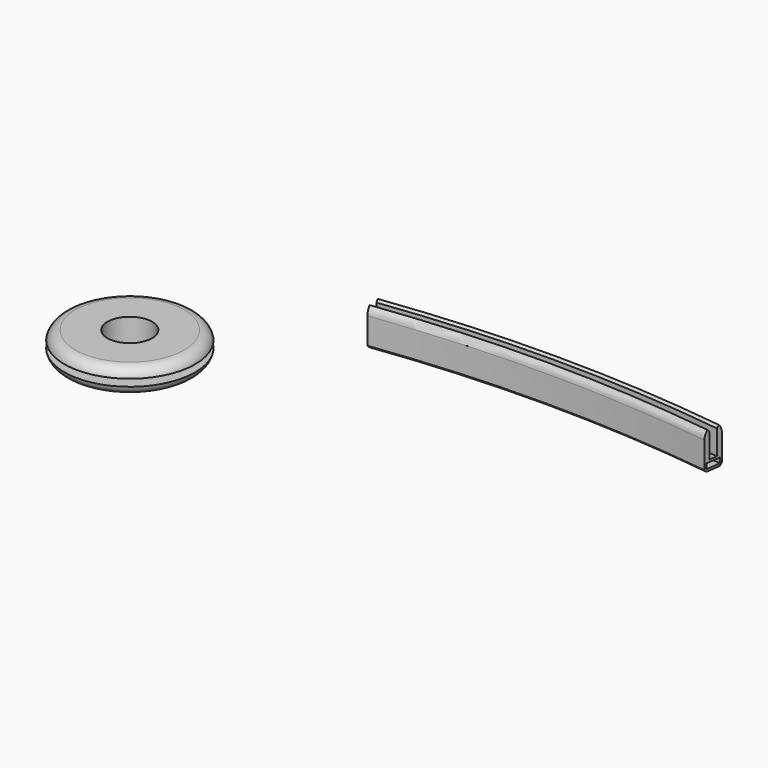
from build123d import *

# Parameters (mm, degrees)
F1_DEPTH    = 1
F4_DEPTH    = 1
F6_DEPTH    = 12
F7_SIZE     = 1
F8_T2_ANGLE = 16.6478295889
F8_T4_ANGLE = 16.6225349948
F11_SIZE    = 1
F12_R       = 22
F12_R_2     = 10
F13_DEPTH   = 3.175
F14_R       = 29.2671438264
F15_DEPTH   = 4
F17_DEPTH   = 25
F18_R       = 29.2671438264
F18_R_2     = 10
F19_DEPTH   = 4
F21_R       = 18.8886705246
F21_R_2     = 17.8886705246
F22_DEPTH   = 8


# Not quite as in the source:
# - a fillet or chamfer that OpenCascade refuses, or shapes differently, is made with other operations: its cross-section is extruded or revolved along the edge and cut away or added


with BuildPart() as f1:
    # F0 (on Top) → F1 (new body)
    with BuildSketch(Plane.XY):
        Polygon((76.2, -1.75), (76.2, 1.75), (76.2, 6.1025535688), (-76.2, 6.1025535688), (-76.2, 1.75), (-76.2, -1.75), (-76.2, -6.1025535688), (76.2, -6.1025535688), align=None)
    extrude(amount=-F1_DEPTH)


with BuildPart() as f4:
    # F3 (on Top) → F4 (new body)
    with BuildSketch(Plane.XY):
        with BuildLine():
            Line((76.2692624922, -4.1994154081), (76.5932074415, -1.7204923214))
            ThreePointArc((76.5932074415, -1.7204923214), (0.8467303705, 3.2078201362), (-74.8997467005, -1.7204923214))
            Line((-74.8997467005, -1.7204923214), (-74.5758017512, -4.1994154081))
            ThreePointArc((-74.5758017512, -4.1994154081), (0.8467303705, 0.7078201362), (76.2692624922, -4.1994154081))
        make_face()
        with BuildLine():
            Line((76.5932074415, -1.7204923214), (77.0467303705, 1.75))
            ThreePointArc((77.0467303705, 1.75), (0.8467303705, 6.7078201362), (-75.3532696295, 1.75))
            Line((-75.3532696295, 1.75), (-74.8997467005, -1.7204923214))
            ThreePointArc((-74.8997467005, -1.7204923214), (0.8467303705, 3.2078201362), (76.5932074415, -1.7204923214))
        make_face()
        with BuildLine():
            ThreePointArc((-75.3532696295, 1.75), (0.8467303705, 6.7078201362), (77.0467303705, 1.75))
            Line((77.0467303705, 1.75), (77.3706753198, 4.2289230867))
            ThreePointArc((77.3706753198, 4.2289230867), (0.8467303705, 9.2078201362), (-75.6772145787, 4.2289230867))
            Line((-75.6772145787, 4.2289230867), (-75.3532696295, 1.75))
        make_face()
    extrude(amount=-F4_DEPTH)

    # F5 (on face) → F6 (join)
    with BuildSketch(Plane.XY):
        with BuildLine():
            ThreePointArc((-75.3532696295, 1.75), (0.8467303705, 6.7078201362), (77.0467303705, 1.75))
            Line((77.0467303705, 1.75), (77.3706753198, 4.2289230867))
            ThreePointArc((77.3706753198, 4.2289230867), (0.8467303705, 9.2078201362), (-75.6772145787, 4.2289230867))
            Line((-75.6772145787, 4.2289230867), (-75.3532696295, 1.75))
        make_face()
        with BuildLine():
            Line((76.2692624922, -4.1994154081), (76.5932074415, -1.7204923214))
            ThreePointArc((76.5932074415, -1.7204923214), (0.8467303705, 3.2078201362), (-74.8997467005, -1.7204923214))
            Line((-74.8997467005, -1.7204923214), (-74.5758017512, -4.1994154081))
            ThreePointArc((-74.5758017512, -4.1994154081), (0.8467303705, 0.7078201362), (76.2692624922, -4.1994154081))
        make_face()
    extrude(amount=F6_DEPTH)

    # F7
    f7_edges = [f4.edges().sort_by_distance(p)[0] for p in [
        (0.84673, 6.70782, 12),
        (0.84673, 3.20782, 12),
    ]]
    chamfer(f7_edges, length=F7_SIZE)

    # F8: fillet of radius 5 on 2 edges, made by hand

    # F8_s1 → F8_t2 (revolve, cut)
    with BuildSketch(Plane(origin=(-82.446715332, -12.0628221249, 0), x_dir=(0, 0, 1), z_dir=(-0.9894654498, -0.1447692085, 0))):
        with BuildLine():
            ThreePointArc((12.0001071227, 8.2094487393), (10.36586952, 7.099643712), (8.4293487989, 6.709403738))
            Line((8.4293487989, 6.709403738), (8.4293487989, 6.609403738))
            ThreePointArc((8.4293487989, 6.609403738), (10.2146743994, 6.609553738), (12, 6.609553738))
            Line((12, 6.609553738), (12.1, 6.709553738))
            ThreePointArc((12.1, 6.709553738), (12.1, 7.4595012386), (12.0715222892, 8.1394496393))
            Line((12.0715222892, 8.1394496393), (12.0001071227, 8.2094487393))
        make_face()
    revolve(axis=Axis((0.8467303705, -581.3550603549, 12), (0, 0, -1)), revolution_arc=F8_T2_ANGLE, mode=Mode.SUBTRACT)

    # F8_s3 → F8_t4 (revolve, cut)
    with BuildSketch(Plane(origin=(83.9817821189, -12.2684844413, 0), x_dir=(0, 0, 1), z_dir=(0.9894973816, -0.1445507933, 0))):
        with BuildLine():
            ThreePointArc((8.4293487989, -15.4361160503), (10.36586952, -15.0458760762), (12.0001071227, -13.9360710489))
            Line((12.0001071227, -13.9360710489), (12.0715222892, -14.0060701489))
            ThreePointArc((12.0715222892, -14.0060701489), (12.1, -14.6860185496), (12.1, -15.4359660503))
            Line((12.1, -15.4359660503), (12, -15.5359660503))
            ThreePointArc((12, -15.5359660503), (10.2146743994, -15.5359660503), (8.4293487989, -15.5361160503))
            Line((8.4293487989, -15.5361160503), (8.4293487989, -15.4361160503))
        make_face()
    revolve(axis=Axis((0.8467303705, -581.3550603549, 12), (0, 0, 1)), revolution_arc=F8_T4_ANGLE, mode=Mode.SUBTRACT)

    # F10: sweep along a path in F10_path
    with BuildLine(Plane(origin=(76.2692624922, -4.1994154081, -1), x_dir=(0, -1, 0), z_dir=(0, 0, -1))) as f10_path:
        ThreePointArc((0, 0), (-4.9072355443, 75.4225321217), (0, 150.8450642434))
    # F9 (on face) → F10 (sweep)
    with BuildSketch(Plane(origin=(-73.8632044186, -9.6524221094, 0), x_dir=(0.1295779797, -0.9915692347, 0), z_dir=(-0.9915692347, -0.1295779797, 0))):
        Polygon((-5.4993706043, -4.3409038335), (-5.4993706043, -1), (-6.4993706043, -1), (-6.4993706043, -3.3409038335), (-12.9993706043, -3.3409038335), (-12.9993706043, -1), (-13.9993706043, -1), (-13.9993706043, -4.3409038335), align=None)
    sweep(path=f10_path.line)

    # F11
    f11_edges = [f4.edges().sort_by_distance(p)[0] for p in [
        (0.84673, 0.70782, -4.340904),
        (0.84673, 9.20782, -4.340904),
    ]]
    chamfer(f11_edges, length=F11_SIZE)


with BuildPart() as f13:
    # F12 (on Top) → F13 (new body)
    with BuildSketch(Plane.XY):
        with Locations((-134.2629939318, -62.5356882811)):
            Circle(F12_R)
        with Locations((-134.2629939318, -62.5356882811)):
            Circle(F12_R_2, mode=Mode.SUBTRACT)
    extrude(amount=F13_DEPTH)

    # F14 (on face) → F15 (join)
    with BuildSketch(Plane.XY.offset(3.175)):
        with Locations((-134.2629939318, -62.5356882811)):
            Circle(F14_R)
    extrude(amount=F15_DEPTH)

    # F16: fillet of radius 5 on 1 edges, made by hand

    # F16_s1 → F16_t2 (revolve, cut)
    with BuildSketch(Plane.XZ.offset(62.5356882811)):
        with BuildLine():
            ThreePointArc((-104.9958501054, 3.175), (-106.7325519308, 6.0479833462), (-109.894829591, 7.175))
            Line((-109.894829591, 7.175), (-104.9958501054, 7.175))
            Line((-104.9958501054, 7.175), (-104.9958501054, 3.175))
        make_face()
    revolve(axis=Axis((-134.2629939318, -62.5356882811, 7.175), (0, 0, 1)), mode=Mode.SUBTRACT)

    # F17 (cut): a face of the model
    f17_faces = [f13.faces().sort_by_distance(p)[0] for p in [
        (-134.2629939318, -62.5356882811, 3.175),
    ]]
    extrude(f17_faces, amount=-F17_DEPTH, mode=Mode.SUBTRACT)

    # F18 (on face) → F19 (join)
    with BuildSketch(Plane(origin=(0, 0, 0), x_dir=(1, 0, 0), z_dir=(0, 0, -1))):
        with Locations((-134.2629939318, 62.5356882811)):
            Circle(F18_R)
        with Locations((-134.2629939318, 62.5356882811)):
            Circle(F18_R_2, mode=Mode.SUBTRACT)
    extrude(amount=F19_DEPTH)

    # F20: fillet of radius 5 on 1 edges, made by hand

    # F20_s1 → F20_t2 (revolve, cut)
    with BuildSketch(Plane.XZ.offset(62.5356882811)):
        with BuildLine():
            ThreePointArc((-104.9958501054, 0), (-106.7325519308, -2.8729833462), (-109.894829591, -4))
            Line((-109.894829591, -4), (-104.9958501054, -4))
            Line((-104.9958501054, -4), (-104.9958501054, 0))
        make_face()
    revolve(axis=Axis((-134.2629939318, -62.5356882811, -4), (0, 0, -1)), mode=Mode.SUBTRACT)


with BuildPart() as f22:
    # F21 (on face) → F22 (new body)
    with BuildSketch(Plane(origin=(0, 0, -4), x_dir=(1, 0, 0), z_dir=(0, 0, -1))):
        with Locations((-134.2629939318, 62.5356882811)):
            Circle(F21_R)
        with Locations((-134.2629939318, 62.5356882811)):
            Circle(F21_R_2, mode=Mode.SUBTRACT)
    extrude(amount=-F22_DEPTH)


with BuildPart() as f13_1:
    add(f13.part)

    # F23: cut F22
    add(f22.part, mode=Mode.SUBTRACT)


solid = Compound([f4.part, f22.part, f13_1.part])
